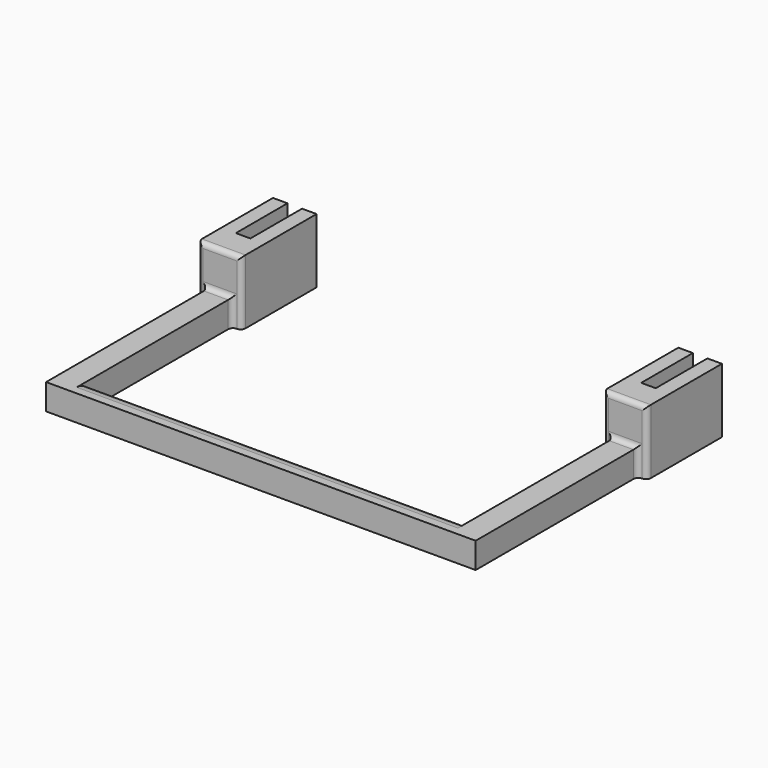
from build123d import *

# Parameters (mm, degrees)
F1_DEPTH    = 8
F3_DEPTH    = 12
F4_R        = 1.5
F5_R        = 1.5
F6_T1_DEPTH = 118.05


# Not quite as in the source:
# - a fillet or chamfer that OpenCascade refuses, or shapes differently, is made with other operations: its cross-section is extruded or revolved along the edge and cut away or added


with BuildPart() as f1:
    # F0 (on Top) → F1 (new body)
    with BuildSketch(Plane.XY):
        Polygon((-127.8, 0), (-132.3, 0), (-132.3, -29), (-129.3, -29), (-129.3, -91.6), (3.75, -91.6), (3.75, -29), (6.75, -29), (6.75, 0), (2.25, 0), (2.25, -20), (-2.25, -20), (-2.25, 0), (-6.75, 0), (-6.75, -29), (-3.75, -29), (-3.75, -84.1), (-121.8, -84.1), (-121.8, -29), (-118.8, -29), (-118.8, 0), (-123.3, 0), (-123.3, -20), (-127.8, -20), align=None)
    extrude(amount=F1_DEPTH)

    # F2 (on face) → F3 (join)
    with BuildSketch(Plane.XY.offset(8)):
        Polygon((-127.8, 0), (-132.3, 0), (-132.3, -29), (-118.8, -29), (-118.8, 0), (-123.3, 0), (-123.3, -20), (-127.8, -20), align=None)
        Polygon((-2.25, 0), (-6.75, 0), (-6.75, -29), (6.75, -29), (6.75, 0), (2.25, 0), (2.25, -20), (-2.25, -20), align=None)
    extrude(amount=F3_DEPTH)

    # F4
    f4_edges = [f1.edges().sort_by_distance(p)[0] for p in [
        (-129.3, -29, 4),
        (-125.55, -29, 8),
        (-121.8, -29, 4),
        (-3.75, -29, 4),
        (0, -29, 8),
        (3.75, -29, 4),
    ]]
    fillet(f4_edges, radius=F4_R)

    # F5
    f5_edges = [f1.edges().sort_by_distance(p)[0] for p in [
        (-132.3, -29, 10),
        (-125.55, -29, 20),
        (-118.8, -29, 10),
        (6.75, -29, 10),
        (0, -29, 20),
        (-6.75, -29, 10),
    ]]
    fillet(f5_edges, radius=F5_R)

    # F6: fillet of radius 5 on 2 edges, made by hand

    # F6_s2 → F6_t1 (cut)
    with BuildSketch(Plane.YZ.offset(-121.8)):
        with BuildLine():
            ThreePointArc((-84.1, 3), (-85.5644660941, 6.5355339059), (-89.1, 8))
            Line((-89.1, 8), (-84.1, 8))
            Line((-84.1, 8), (-84.1, 3))
        make_face()
        with BuildLine():
            ThreePointArc((-89.1, 0), (-85.5644660941, 1.4644660941), (-84.1, 5))
            Line((-84.1, 5), (-84.1, 0))
            Line((-84.1, 0), (-89.1, 0))
        make_face()
    extrude(amount=F6_T1_DEPTH, mode=Mode.SUBTRACT)


solid = f1.part
